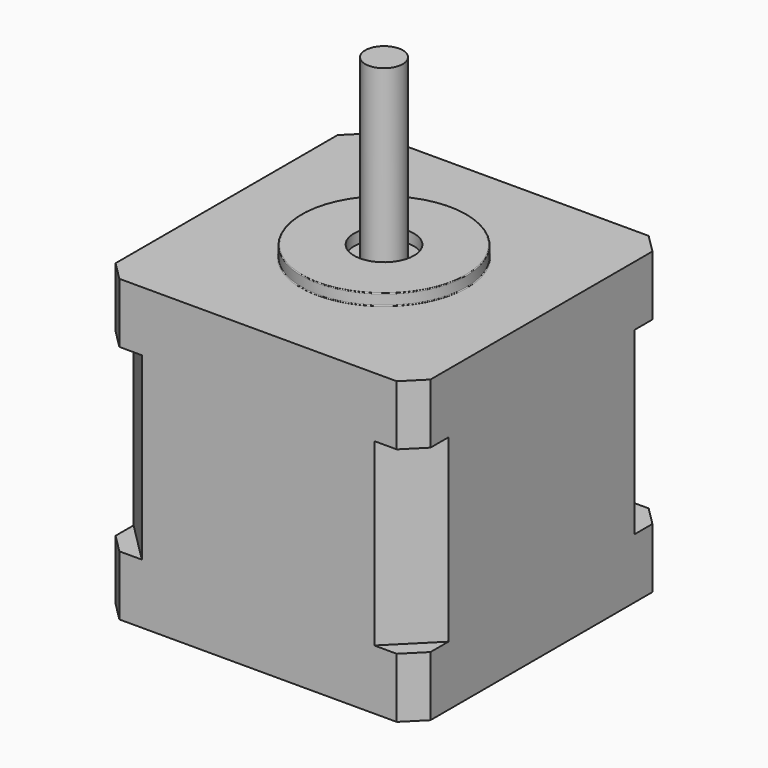
from build123d import *

# Parameters (mm, degrees)
F0_W      = 42
F0_H      = 42
F1_DEPTH  = 8
F2_DEPTH  = 24
F3_DEPTH  = 8
F4_SIZE   = 2.5
F4_2_SIZE = 2.5
F5_SIZE   = 5.5
F7_R      = 11
F7_R_2    = 4
F8_DEPTH  = 1.5
F9_R      = 2.5
F10_DEPTH = 23.5
F12_R     = 0.1


# Not quite as in the source:
# - a feature names something its author has since deleted; it is built from what else it names


with BuildPart() as f1:
    # F0 (on Top) → F1 (new body)
    with BuildSketch(Plane.XY):
        Rectangle(F0_W, F0_H)
    extrude(amount=F1_DEPTH)


with BuildPart() as f2:
    # F2 (new): a face of the model
    f2_faces = [f1.part.faces().sort_by_distance(p)[0] for p in [
        (0, 0, 8),
    ]]
    extrude(f2_faces, amount=F2_DEPTH)


with BuildPart() as f3:
    # F3 (new): a face of the model
    f3_faces = [f2.part.faces().sort_by_distance(p)[0] for p in [
        (0, 0, 32),
    ]]
    extrude(f3_faces, amount=F3_DEPTH)

    # F4#2
    f4_2_edges = [f3.edges().sort_by_distance(p)[0] for p in [
        (-21, -21, 36),
        (-21, 21, 36),
        (21, 21, 36),
        (21, -21, 36),
    ]]
    chamfer(f4_2_edges, length=F4_2_SIZE)

    # F7 (on face) → F8 (join)
    with BuildSketch(Plane.XY.offset(40)):
        Circle(F7_R)
        Circle(F7_R_2, mode=Mode.SUBTRACT)
    extrude(amount=F8_DEPTH)

    # F9 (on face) → F10 (join)
    with BuildSketch(Plane.XY.offset(40)):
        Circle(F9_R)
    extrude(amount=F10_DEPTH)


with BuildPart() as f1_1:
    add(f1.part)

    # F4
    f4_edges = [f1_1.edges().sort_by_distance(p)[0] for p in [
        (-21, -21, 4),
        (-21, 21, 4),
        (21, 21, 4),
        (21, -21, 4),
    ]]
    chamfer(f4_edges, length=F4_SIZE)


with BuildPart() as f2_1:
    add(f2.part)

    # F5
    f5_edges = [f2_1.edges().sort_by_distance(p)[0] for p in [
        (21, -21, 20),
        (-21, -21, 20),
        (-21, 21, 20),
        (21, 21, 20),
    ]]
    chamfer(f5_edges, length=F5_SIZE)


with BuildPart() as f1_2:
    add(f1_1.part)

    # F11: union F2, F3
    add(f2_1.part)
    add(f3.part)

    # F12
    f12_edges = [f1_2.edges().sort_by_distance(p)[0] for p in [
        (11, 0, 40.75),
        (-11, 0, 40),
        (-11, 0, 41.5),
    ]]
    fillet(f12_edges, radius=F12_R)


solid = f1_2.part
